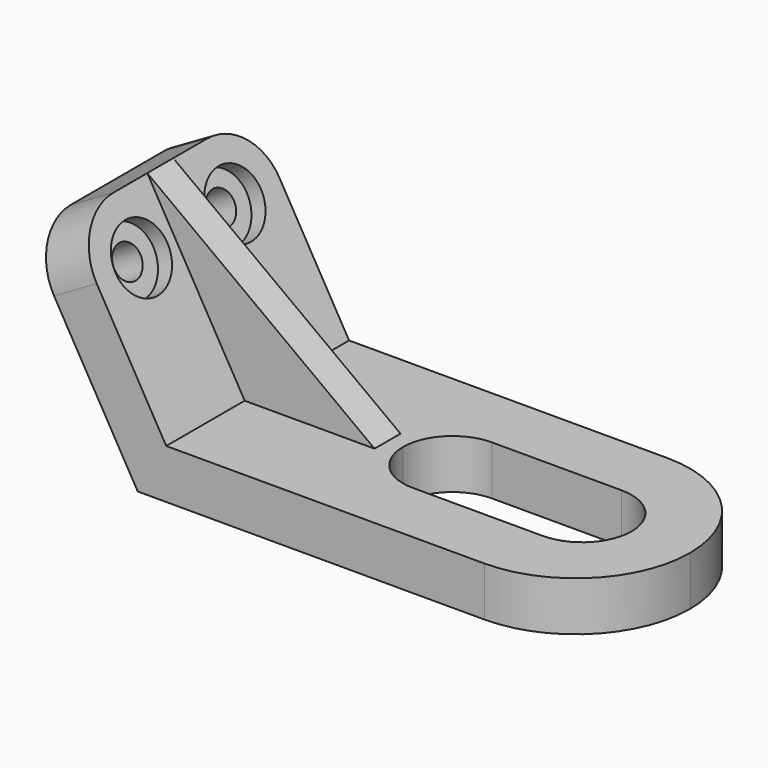
from build123d import *

# Parameters (mm, degrees)
F1_DEPTH  = 22.352
F2_DEPTH  = 3.175
F4_DEPTH  = 1143
F6_R      = 6.35
F6_R_2    = 3.175
F7_DEPTH  = 3.175
F8_R      = 6.35
F8_R_2    = 3.175
F9_DEPTH  = 3.175
F10_DEPTH = 28.5637839421
F11_R     = 10.922
F12_R     = 22.35199


# Not quite as in the source:
# - a fillet or chamfer is up to 0.001 mm smaller than in the source, because OpenCascade refuses the exact size


with BuildPart() as f1:
    # F0 (on Front) → F1 (new body, symmetric)
    with BuildSketch(Plane.XZ):
        Polygon((-14.5947370299, 9.652), (-33.6447370299, 42.6475678842), (-42.0036142272, 37.8215678842), (-20.1673218281, 0), (69.9872629701, 0), (69.9872629701, 9.652), (10.8052629701, 9.652), align=None)
    extrude(amount=F1_DEPTH, both=True)

    # F0 (on Front) → F2 (join, symmetric)
    with BuildSketch(Plane.XZ):
        Polygon((10.8052629701, 9.652), (-33.6447370299, 42.6475678842), (-14.5947370299, 9.652), align=None)
    extrude(amount=F2_DEPTH, both=True)

    # F3 (on face) → F4 (cut)
    with BuildSketch(Plane.XY.offset(9.652)):
        with BuildLine():
            ThreePointArc((23.5052629701, 9.652), (16.6802683181, 6.824994652), (13.8532629701, 0))
            Line((13.8532629701, 0), (23.5052629701, 0))
            Line((23.5052629701, 0), (26.5532629701, 0))
            ThreePointArc((26.5532629701, 0), (27.1079902762, 4.9488187589), (28.7446379798, 9.652))
            Line((28.7446379798, 9.652), (23.5052629701, 9.652))
        make_face()
        with BuildLine():
            Line((23.5052629701, 0), (13.8532629701, 0))
            ThreePointArc((13.8532629701, 0), (16.6802683181, -6.824994652), (23.5052629701, -9.652))
            Line((23.5052629701, -9.652), (28.7446379798, -9.652))
            ThreePointArc((28.7446379798, -9.652), (27.1079902762, -4.9488187589), (26.5532629701, 0))
            Line((26.5532629701, 0), (23.5052629701, 0))
        make_face()
        with BuildLine():
            ThreePointArc((28.7446379798, 9.652), (27.1079902762, 4.9488187589), (26.5532629701, 0))
            ThreePointArc((26.5532629701, 0), (27.1079902762, -4.9488187589), (28.7446379798, -9.652))
            Line((28.7446379798, -9.652), (48.9052629701, -9.652))
            ThreePointArc((48.9052629701, -9.652), (58.5572629701, 0), (48.9052629701, 9.652))
            Line((48.9052629701, 9.652), (28.7446379798, 9.652))
        make_face()
    extrude(amount=-F4_DEPTH, mode=Mode.SUBTRACT)

    # F6 (on face) → F7 (cut)
    with BuildSketch(Plane(origin=(-6.7666141738, 0, -3.9067065147), x_dir=(0, 1, 0), z_dir=(0.8660254038, 0, 0.5))):
        with Locations((11.43, 42.8342457123)):
            Circle(F6_R)
        with Locations((11.43, 42.8342457123)):
            Circle(F6_R_2, mode=Mode.SUBTRACT)
    extrude(amount=-F7_DEPTH, mode=Mode.SUBTRACT)

    # F8 (on face) → F9 (cut)
    with BuildSketch(Plane(origin=(-6.7666141738, 0, -3.9067065147), x_dir=(0, 1, 0), z_dir=(0.8660254038, 0, 0.5))):
        with Locations((-11.43, 42.8342457123)):
            Circle(F8_R)
        with Locations((-11.43, 42.8342457123)):
            Circle(F8_R_2, mode=Mode.SUBTRACT)
    extrude(amount=-F9_DEPTH, mode=Mode.SUBTRACT)

    # F10 (cut, through all): faces of the model
    f10_faces = [f1.faces().sort_by_distance(p)[0] for p in [
        (-28.1837370299, -11.43, 33.1888384241),
        (-28.1837370299, 11.43, 33.1888384241),
    ]]
    extrude(f10_faces, amount=-F10_DEPTH, mode=Mode.SUBTRACT)

    # F11
    f11_edges = [f1.edges().sort_by_distance(p)[0] for p in [
        (-37.824176, -22.352, 40.234568),
        (-37.824176, 22.352, 40.234568),
    ]]
    fillet(f11_edges, radius=F11_R)

    # F12 (radius 22.352 in the source; OpenCascade refuses exactly that, so slightly less here)
    f12_edges = [f1.edges().sort_by_distance(p)[0] for p in [
        (69.987263, 22.352, 4.826),
        (69.987263, -22.352, 4.826),
    ]]
    fillet(f12_edges, radius=F12_R)


solid = f1.part
